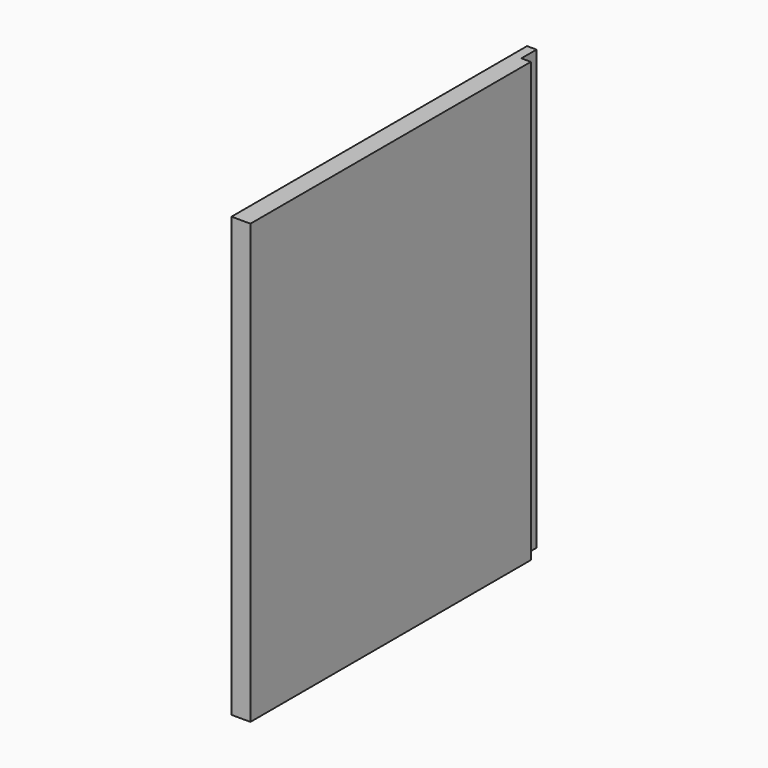
from build123d import *

# Parameters (mm, degrees)
F0_W     = 234.95
F0_H     = 279.4
F2_DEPTH = 12.065
F3_W     = 12.065
F3_H     = 279.4
F4_DEPTH = 6.0325
F5_DEPTH = 0.4445


# Not quite as in the source:
# - a variable given as a bare number and used for a length is read in inches; the dataset says mm whatever the document's units were


with BuildPart() as f2:
    # F0 (on Right) → F2 (new body)
    with BuildSketch(Plane.YZ):
        Rectangle(F0_W, F0_H)
    extrude(amount=F2_DEPTH)

    # F3 (on face) → F4 (cut)
    with BuildSketch(Plane.YZ.offset(12.065)):
        with Locations((111.4425, 0)):
            Rectangle(F3_W, F3_H)
    extrude(amount=-F4_DEPTH, mode=Mode.SUBTRACT)

    # F5 (cut): a face of the model
    f5_faces = [f2.faces().sort_by_distance(p)[0] for p in [
        (5.9530149098, -2.9367649098, 139.7),
    ]]
    extrude(f5_faces, amount=-F5_DEPTH, mode=Mode.SUBTRACT)


solid = f2.part
